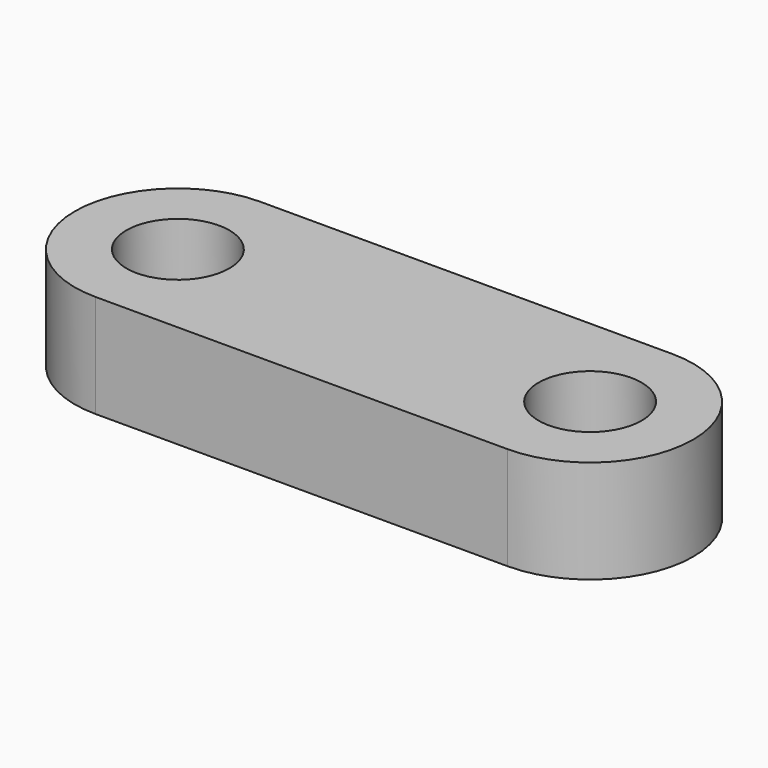
from build123d import *

# Parameters (mm, degrees)
F2_DEPTH = 12.7
F3_R     = 6.35
F4_DEPTH = 12.701


# Not quite as in the source:
# - a variable given as a bare number and used for a length is read in inches; the dataset says mm whatever the document's units were


with BuildPart() as f2:
    # F1 (on Top) → F2 (new body)
    with BuildSketch(Plane.XY):
        with BuildLine():
            Line((-50.8, -12.7), (0, -12.7))
            ThreePointArc((0, -12.7), (12.7, 0), (0, 12.7))
            Line((0, 12.7), (-50.8, 12.7))
            ThreePointArc((-50.8, 12.7), (-63.5, 0), (-50.8, -12.7))
        make_face()
    extrude(amount=F2_DEPTH)

    # F3 (on face) → F4 (cut, through all)
    with BuildSketch(Plane.XY.offset(12.7)):
        Circle(F3_R)
        with Locations((-50.8, 0)):
            Circle(F3_R)
    extrude(amount=-F4_DEPTH, mode=Mode.SUBTRACT)


solid = f2.part
